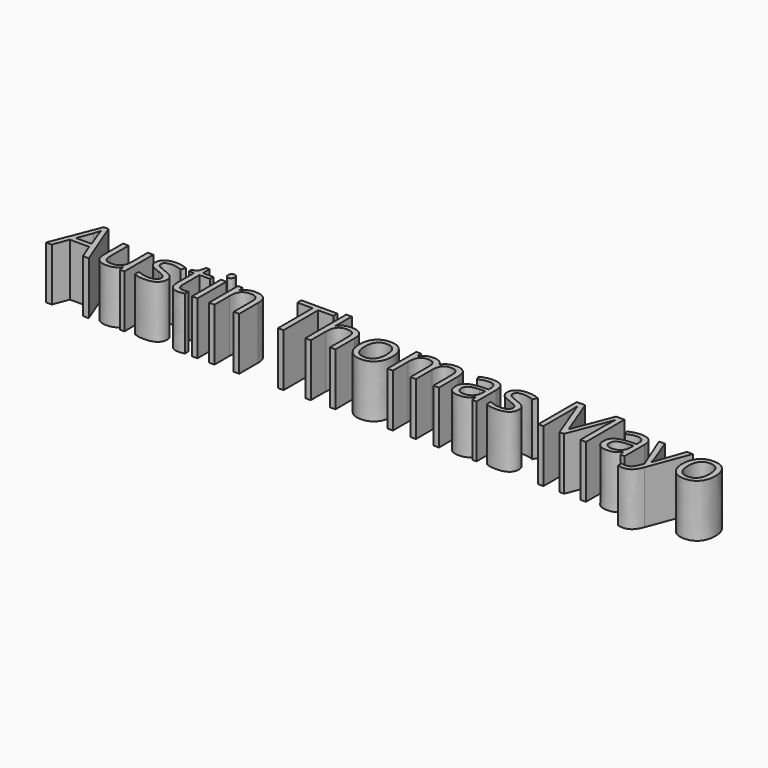
from build123d import *

# Parameters (mm, degrees)
F0_TEXT_SIZE = 9.7352493968
F1_DEPTH     = 7.62


# Not quite as in the source:
# - Text() gives the source's letters only with a copy of the font that has no kerning and outlines rounded to 1/6400 em; it was checked with that copy


with BuildPart() as f1:
    # F0 (on Top) → F1 (new body)
    with BuildSketch(Plane.XY):
        with Locations((-72.2443833947, 40.2242727578)):
            Text('Austin Thomas Mayo', F0_TEXT_SIZE, font='Open Sans', text_align=(TextAlign.LEFT, TextAlign.BOTTOM))
    extrude(amount=F1_DEPTH)


solid = f1.part
